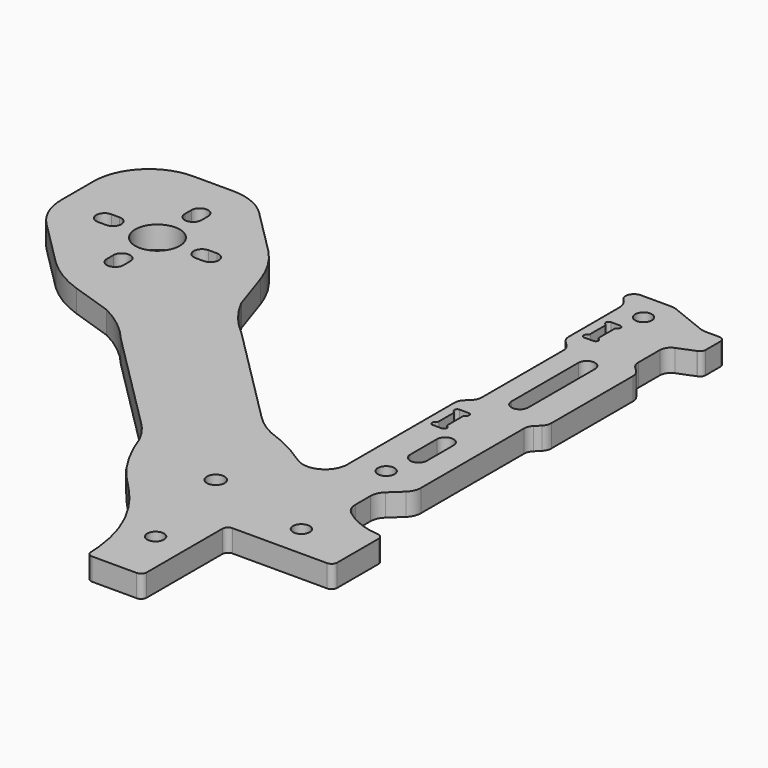
from build123d import *

# Parameters (mm, degrees)
F0_R     = 1.5
F0_R_2   = 1.6
F0_R_3   = 4
F1_DEPTH = 4


# Not quite as in the source:
# - ends of sketch curves that miss each other by under 0.0002 mm in the source are joined


with BuildPart() as f1:
    # F0 (on Top) → F1 (new body)
    with BuildSketch(Plane.XY):
        with BuildLine():
            ThreePointArc((-68.7198979633, -19.2310683136), (-69.2667474289, -19.0706292261), (-69.8340699923, -19.0164983863))
            Line((-69.8340699923, -19.0164983863), (-75.2563229923, -19.0164983863))
            ThreePointArc((-75.2563229923, -19.0164983863), (-76.6575815321, -19.9812652551), (-76.2563229867, -21.63453238))
            ThreePointArc((-76.2563229867, -21.63453238), (-75.5177102079, -22.645855508), (-75.2563229923, -23.8706003863))
            Line((-75.2563229923, -23.8706003863), (-75.2563229923, -35.1880713863))
            ThreePointArc((-75.2563229923, -35.1880713863), (-75.1040821926, -35.9534379244), (-74.6705370547, -36.6022844487))
            Line((-74.6705370547, -36.6022844487), (-73.8421089923, -37.4307123863))
            ThreePointArc((-73.8421089923, -37.4307123863), (-73.408563792, -38.0795588482), (-73.2563229923, -38.8449253863))
            Line((-73.2563229923, -38.8449253863), (-73.2563229923, -57.1880713863))
            ThreePointArc((-73.2563229923, -57.1880713863), (-73.408563792, -57.9534379244), (-73.8421089299, -58.6022844487))
            Line((-73.8421089299, -58.6022844487), (-74.6705369923, -59.4307123863))
            ThreePointArc((-74.6705369923, -59.4307123863), (-75.1040821926, -60.0795588482), (-75.2563229923, -60.8449253863))
            Line((-75.2563229923, -60.8449253863), (-75.2563229923, -84.8364823863))
            ThreePointArc((-75.2563229923, -84.8364823863), (-77.3940816238, -88.3765469458), (-81.5223515351, -88.1327097212))
            ThreePointArc((-81.5223515351, -88.1327097212), (-85.5001057777, -85.7657105269), (-89.7529047165, -83.9384406075))
            ThreePointArc((-89.7529047165, -83.9384406075), (-91.8824323761, -82.6525966161), (-93.7563230573, -81.0164984487))
            Line((-93.7563230573, -81.0164984487), (-111.8499919923, -62.9020143863))
            ThreePointArc((-111.8499919923, -62.9020143863), (-115.0500186095, -59.6637600428), (-117.5068461048, -55.8309464428))
            Line((-117.5068461048, -55.8309464428), (-119.9817199923, -48.4063253863))
            ThreePointArc((-119.9817199923, -48.4063253863), (-121.7314401326, -44.6478315667), (-124.2243601054, -41.3352574916))
            Line((-124.2243601054, -41.3352574916), (-132.7096419923, -32.8499763863))
            ThreePointArc((-132.7096419923, -32.8499763863), (-135.9638712469, -30.7325010032), (-139.7807099968, -30.0215490151))
            Line((-139.7807099968, -30.0215490151), (-146.8517769923, -30.0215493863))
            ThreePointArc((-146.8517769923, -30.0215493863), (-153.8517770371, -32.9210443415), (-156.7512719923, -39.9210443863))
            Line((-156.7512719923, -39.9210443863), (-156.7512719923, -46.9921113863))
            ThreePointArc((-156.7512719923, -46.9921113863), (-156.0403203754, -50.8089501317), (-153.9228453387, -54.0631797243))
            Line((-153.9228453387, -54.0631797243), (-145.4375639923, -62.5484613863))
            ThreePointArc((-145.4375639923, -62.5484613863), (-142.1249898119, -65.0413812461), (-138.3664962297, -66.7911020771))
            Line((-138.3664962297, -66.7911020771), (-130.9418749923, -69.2659753863))
            ThreePointArc((-130.9418749923, -69.2659753863), (-127.1090613358, -71.7228027691), (-123.870807081, -74.922829459))
            Line((-123.870807081, -74.922829459), (-105.8395839923, -92.9540523863))
            ThreePointArc((-105.8395839923, -92.9540523863), (-104.1591231129, -94.8555234649), (-102.8343796027, -97.0199161923))
            ThreePointArc((-102.8343796027, -97.0199161923), (-101.008160191, -101.2706562812), (-98.6427303315, -105.2466606194))
            ThreePointArc((-98.6427303315, -105.2466606194), (-97.1356962685, -107.0614279538), (-95.5198284171, -108.7800038111))
            ThreePointArc((-95.5198284171, -108.7800038111), (-93.1084062482, -111.4552655604), (-90.9867028572, -114.3656532981))
            ThreePointArc((-90.9867028572, -114.3656532981), (-88.2033345479, -120.0250091818), (-86.8576764091, -126.1865554256))
            ThreePointArc((-86.8576764091, -126.1865554256), (-86.7844945691, -127.1166669837), (-86.7401234624, -128.0485974014))
            ThreePointArc((-86.7401234624, -128.0485974014), (-86.436304493, -128.7348642479), (-85.7406389923, -129.0164983863))
            Line((-85.7406389923, -129.0164983863), (-77.7563229923, -129.0164983863))
            ThreePointArc((-77.7563229923, -129.0164983863), (-77.0492162111, -128.7236051675), (-76.7563229923, -128.0164983863))
            Line((-76.7563229923, -128.0164983863), (-76.7563229923, -111.0164983863))
            ThreePointArc((-76.7563229923, -111.0164983863), (-76.4634297735, -110.3093916051), (-75.7563229923, -110.0164983863))
            Line((-75.7563229923, -110.0164983863), (-58.7563229923, -110.0164983863))
            ThreePointArc((-58.7563229923, -110.0164983863), (-58.0492162111, -109.7236051675), (-57.7563229923, -109.0164983863))
            Line((-57.7563229923, -109.0164983863), (-57.7563229923, -99.7079493863))
            ThreePointArc((-57.7563229923, -99.7079493863), (-58.0239146277, -99.02708377), (-58.6834789671, -98.7106060412))
            ThreePointArc((-58.6834789671, -98.7106060412), (-62.3444302283, -97.8887041809), (-65.6066667986, -96.0350861391))
            ThreePointArc((-65.6066667986, -96.0350861391), (-66.4536393859, -94.9868785913), (-66.7563229923, -93.6736823863))
            Line((-66.7563229923, -93.6736823863), (-66.7563229923, -90.3204613863))
            ThreePointArc((-66.7563229923, -90.3204613863), (-66.507662318, -89.1245801569), (-65.8029017157, -88.1269446827))
            Line((-65.8029017157, -88.1269446827), (-63.7097439923, -86.1740013863))
            ThreePointArc((-63.7097439923, -86.1740013863), (-63.0049835307, -85.1763663029), (-62.7563229923, -83.9804853863))
            Line((-62.7563229923, -83.9804853863), (-62.7563229923, -60.8449253863))
            ThreePointArc((-62.7563229923, -60.8449253863), (-62.6040821926, -60.0795588482), (-62.1705370547, -59.4307123239))
            Line((-62.1705370547, -59.4307123239), (-61.3421089923, -58.6022843863))
            ThreePointArc((-61.3421089923, -58.6022843863), (-60.908563792, -57.9534379244), (-60.7563229923, -57.1880713863))
            Line((-60.7563229923, -57.1880713863), (-60.7563229923, -38.8449253863))
            ThreePointArc((-60.7563229923, -38.8449253863), (-60.908563792, -38.0795588482), (-61.3421089299, -37.4307123239))
            Line((-61.3421089299, -37.4307123239), (-62.1705369923, -36.6022843863))
            ThreePointArc((-62.1705369923, -36.6022843863), (-62.6040821926, -35.9534379244), (-62.7563229923, -35.1880713863))
            Line((-62.7563229923, -35.1880713863), (-62.7563229923, -30.3705643863))
            ThreePointArc((-62.7563229923, -30.3705643863), (-62.4124574012, -29.2493066908), (-61.4991041726, -28.5136109355))
            Line((-61.4991041726, -28.5136109355), (-58.4991039923, -27.3136113863))
            ThreePointArc((-58.4991039923, -27.3136113863), (-58.4597438323, -27.2980862298), (-58.4200540366, -27.2834242622))
            ThreePointArc((-58.4200540366, -27.2834242622), (-57.938928047, -26.9177360749), (-57.7563229923, -26.3416583863))
            Line((-57.7563229923, -26.3416583863), (-57.7563229923, -23.0164983863))
            ThreePointArc((-57.7563229923, -23.0164983863), (-58.0492162111, -22.3093916051), (-58.7563229923, -22.0164983863))
            Line((-58.7563229923, -22.0164983863), (-61.1785759923, -22.0164983863))
            ThreePointArc((-61.1785759923, -22.0164983863), (-61.7458985558, -21.9623675465), (-62.2927480214, -21.8019284589))
            Line((-62.2927480214, -21.8019284589), (-68.7198979633, -19.2310683136))
        make_face()
        with Locations((-82.5810189923, -118.7347053863)):
            Circle(F0_R, mode=Mode.SUBTRACT)
        with Locations((-68.0390489923, -104.1927353863)):
            Circle(F0_R, mode=Mode.SUBTRACT)
        with Locations((-86.7563229923, -100.0164983863)):
            Circle(F0_R_2, mode=Mode.SUBTRACT)
        with Locations((-69.7563229923, -83.0164983863)):
            Circle(F0_R, mode=Mode.SUBTRACT)
        with BuildLine():
            Line((-67.2563229923, -71.0164983863), (-67.2563229923, -77.0164983863))
            ThreePointArc((-67.2563229923, -77.0164983863), (-68.7563229923, -78.5164983863), (-70.2563229923, -77.0164983863))
            Line((-70.2563229923, -77.0164983863), (-70.2563229923, -71.0164983863))
            ThreePointArc((-70.2563229923, -71.0164983863), (-68.7563229923, -69.5164983863), (-67.2563229923, -71.0164983863))
        make_face(mode=Mode.SUBTRACT)
        with BuildLine():
            ThreePointArc((-148.5736029923, -49.1992183863), (-150.0736029923, -47.6992183863), (-148.5736029923, -46.1992183863))
            Line((-148.5736029923, -46.1992183863), (-147.0736029923, -46.1992183863))
            ThreePointArc((-147.0736029923, -46.1992183863), (-145.5736029923, -47.6992183863), (-147.0736029923, -49.1992183863))
            Line((-147.0736029923, -49.1992183863), (-148.5736029923, -49.1992183863))
        make_face(mode=Mode.SUBTRACT)
        with BuildLine():
            ThreePointArc((-140.5736029923, -55.6992183863), (-139.0736029923, -54.1992183863), (-137.5736029923, -55.6992183863))
            Line((-137.5736029923, -55.6992183863), (-137.5736029923, -57.1992183863))
            ThreePointArc((-137.5736029923, -57.1992183863), (-139.0736029923, -58.6992183863), (-140.5736029923, -57.1992183863))
            Line((-140.5736029923, -57.1992183863), (-140.5736029923, -55.6992183863))
        make_face(mode=Mode.SUBTRACT)
        with Locations((-139.0736029923, -47.6992183863)):
            Circle(F0_R_3, mode=Mode.SUBTRACT)
        with BuildLine():
            ThreePointArc((-131.0736029923, -49.1992183863), (-132.5736029923, -47.6992183863), (-131.0736029923, -46.1992183863))
            Line((-131.0736029923, -46.1992183863), (-129.5736029923, -46.1992183863))
            ThreePointArc((-129.5736029923, -46.1992183863), (-128.0736029923, -47.6992183863), (-129.5736029923, -49.1992183863))
            Line((-129.5736029923, -49.1992183863), (-131.0736029923, -49.1992183863))
        make_face(mode=Mode.SUBTRACT)
        with BuildLine():
            ThreePointArc((-140.5736029923, -38.1992183863), (-139.0736029923, -36.6992183863), (-137.5736029923, -38.1992183863))
            Line((-137.5736029923, -38.1992183863), (-137.5736029923, -39.6992183863))
            ThreePointArc((-137.5736029923, -39.6992183863), (-139.0736029923, -41.1992183863), (-140.5736029923, -39.6992183863))
            Line((-140.5736029923, -39.6992183863), (-140.5736029923, -38.1992183863))
        make_face(mode=Mode.SUBTRACT)
        with BuildLine():
            Line((-73.4063229923, -62.0164983863), (-71.7563229923, -62.0164983863))
            ThreePointArc((-71.7563229923, -62.0164983863), (-71.2733600599, -62.3870889357), (-71.5063231214, -62.9495111627))
            ThreePointArc((-71.5063231214, -62.9495111627), (-71.689335782, -63.1325235382), (-71.7563229923, -63.3825233863))
            Line((-71.7563229923, -63.3825233863), (-71.7563229923, -66.6504733863))
            ThreePointArc((-71.7563229923, -66.6504733863), (-71.689335782, -66.9004732343), (-71.5063232963, -67.0834859127))
            ThreePointArc((-71.5063232963, -67.0834859127), (-71.2733600599, -67.6459078368), (-71.7563229923, -68.0164983863))
            Line((-71.7563229923, -68.0164983863), (-73.4063229923, -68.0164983863))
            ThreePointArc((-73.4063229923, -68.0164983863), (-73.8892859248, -67.6459078368), (-73.6563228632, -67.0834856099))
            ThreePointArc((-73.6563228632, -67.0834856099), (-73.4733102027, -66.9004732343), (-73.4063229923, -66.6504733863))
            Line((-73.4063229923, -66.6504733863), (-73.4063229923, -63.3825233863))
            ThreePointArc((-73.4063229923, -63.3825233863), (-73.4733102027, -63.1325235382), (-73.6563226884, -62.9495108599))
            ThreePointArc((-73.6563226884, -62.9495108599), (-73.8892859248, -62.3870889357), (-73.4063229923, -62.0164983863))
        make_face(mode=Mode.SUBTRACT)
        with BuildLine():
            Line((-66.2563229923, -40.5164983863), (-66.2563229923, -55.5164983863))
            ThreePointArc((-66.2563229923, -55.5164983863), (-67.7563229923, -57.0164983863), (-69.2563229923, -55.5164983863))
            Line((-69.2563229923, -55.5164983863), (-69.2563229923, -40.5164983863))
            ThreePointArc((-69.2563229923, -40.5164983863), (-67.7563229923, -39.0164983863), (-66.2563229923, -40.5164983863))
        make_face(mode=Mode.SUBTRACT)
        with BuildLine():
            Line((-73.4063229923, -28.0164983863), (-71.7563229923, -28.0164983863))
            ThreePointArc((-71.7563229923, -28.0164983863), (-71.2733600599, -28.3870889357), (-71.5063231214, -28.9495111627))
            ThreePointArc((-71.5063231214, -28.9495111627), (-71.689335782, -29.1325235382), (-71.7563229923, -29.3825233863))
            Line((-71.7563229923, -29.3825233863), (-71.7563229923, -32.6504733863))
            ThreePointArc((-71.7563229923, -32.6504733863), (-71.689335782, -32.9004732343), (-71.5063232963, -33.0834859127))
            ThreePointArc((-71.5063232963, -33.0834859127), (-71.2733600599, -33.6459078368), (-71.7563229923, -34.0164983863))
            Line((-71.7563229923, -34.0164983863), (-73.4063229923, -34.0164983863))
            ThreePointArc((-73.4063229923, -34.0164983863), (-73.8892859248, -33.6459078368), (-73.6563228632, -33.0834856099))
            ThreePointArc((-73.6563228632, -33.0834856099), (-73.4733102027, -32.9004732343), (-73.4063229923, -32.6504733863))
            Line((-73.4063229923, -32.6504733863), (-73.4063229923, -29.3825233863))
            ThreePointArc((-73.4063229923, -29.3825233863), (-73.4733102027, -29.1325235382), (-73.6563226884, -28.9495108599))
            ThreePointArc((-73.6563226884, -28.9495108599), (-73.8892859248, -28.3870889357), (-73.4063229923, -28.0164983863))
        make_face(mode=Mode.SUBTRACT)
        with Locations((-70.7563229923, -24.0164983863)):
            Circle(F0_R, mode=Mode.SUBTRACT)
    extrude(amount=F1_DEPTH)


solid = f1.part
